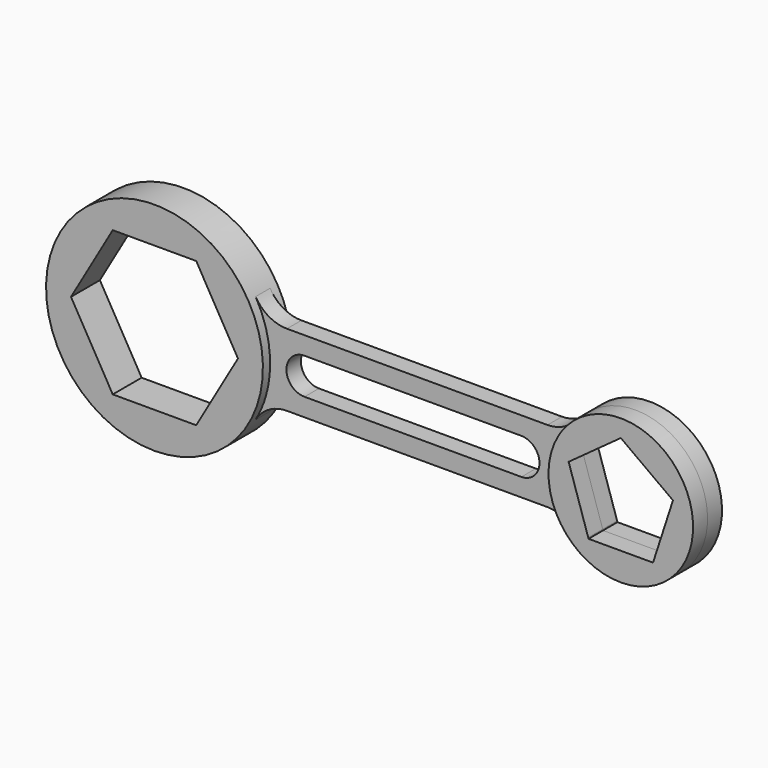
from build123d import *

# Parameters (mm, degrees)
F1_DEPTH = 127
F2_DEPTH = 63.5


with BuildPart() as f1:
    # F0 (on Front) → F1 (new body, symmetric)
    with BuildSketch(Plane.XZ):
        with BuildLine():
            ThreePointArc((-343.3886423163, -254), (-267.2645203677, -70.2201123681), (-241.3, 127))
            ThreePointArc((-241.3, 127), (-267.2645203677, 324.2201123681), (-343.3886423163, 508))
            ThreePointArc((-343.3886423163, 508), (-1765.3, 127), (-343.3886423163, -254))
        make_face()
        Polygon((-416.7121265033, 127), (-710.0060632517, -381), (-1296.5939367483, -381), (-1589.8878734967, 127), (-1296.5939367483, 635), (-710.0060632517, 635), align=None, mode=Mode.SUBTRACT)
    extrude(amount=F1_DEPTH, both=True)


with BuildPart() as f1b:
    # F0 (on Front) → F1, piece 2 (new body, symmetric)
    with BuildSketch(Plane.XZ):
        with BuildLine():
            ThreePointArc((2781.2957251752, 124.6933945575), (2455.5263714034, 598.8832210777), (1896.0359158238, 464.8977981858))
            ThreePointArc((1896.0359158238, 464.8977981858), (1863.2140679876, 424.521736177), (1834.6946262179, 381))
            ThreePointArc((1834.6946262179, 381), (1767.7537116518, 74.7807452315), (1893.2850874873, -212.4355351475))
            ThreePointArc((1893.2850874873, -212.4355351475), (2453.599075192, -350.2326017543), (2781.2957251752, 124.6933945575))
        make_face()
        Polygon((2273.2957251752, 510.157635163), (2279.5099828097, 505.6427127116), (2633.6797453674, 248.3233180798), (2639.8940030018, 243.8083956284), (2637.5203678003, 236.5030976454), (2502.2395562907, -179.8484288332), (2499.8659210892, -187.1537268162), (2492.1846762233, -187.1537268162), (2054.4067741271, -187.1537268162), (2046.7255292612, -187.1537268162), (2044.3518940597, -179.8484288332), (1909.0710825501, 236.5030976455), (1906.6974473486, 243.8083956284), (1912.911704983, 248.3233180798), (2267.0814675408, 505.6427127116), align=None, mode=Mode.SUBTRACT)
    extrude(amount=F1_DEPTH, both=True)


with BuildPart() as f2:
    # F0 (on Front) → F2 (new body, symmetric)
    with BuildSketch(Plane.XZ):
        with BuildLine():
            ThreePointArc((-343.3886423163, 508), (-267.2645203677, 324.2201123681), (-241.3, 127))
            ThreePointArc((-241.3, 127), (-267.2645203677, -70.2201123681), (-343.3886423163, -254))
            ThreePointArc((-343.3886423163, -254), (-250.418189755, -161.0295474388), (-123.418189755, -127))
            Line((-123.418189755, -127), (1651, -127))
            Line((1651, -127), (1703.2797686434, -127))
            ThreePointArc((1703.2797686434, -127), (1807.4446041865, -149.3414429893), (1893.2850874873, -212.4355351475))
            ThreePointArc((1893.2850874873, -212.4355351475), (1767.7537116518, 74.7807452315), (1834.6946262179, 381))
            ThreePointArc((1834.6946262179, 381), (1863.2140679876, 424.521736177), (1896.0359158238, 464.8977981858))
            ThreePointArc((1896.0359158238, 464.8977981858), (1810.6291692551, 402.920316205), (1707.406011148, 381))
            Line((1707.406011148, 381), (1651, 381))
            Line((1651, 381), (-123.418189755, 381))
            ThreePointArc((-123.418189755, 381), (-250.418189755, 415.0295474388), (-343.3886423163, 508))
        make_face()
        with BuildLine():
            Line((1524, 0), (0, 0))
            ThreePointArc((0, 0), (-127, 127), (0, 254))
            Line((0, 254), (1524, 254))
            ThreePointArc((1524, 254), (1651, 127), (1524, 0))
        make_face(mode=Mode.SUBTRACT)
    extrude(amount=F2_DEPTH, both=True)


solid = Compound([f1.part, f1b.part, f2.part])
